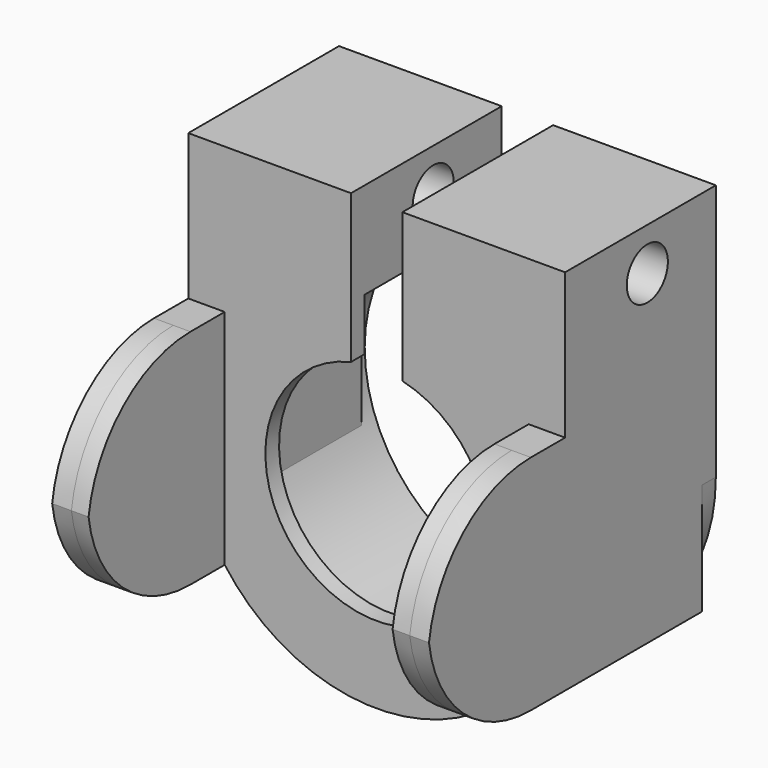
from build123d import *
from build123d import SkipClean  # not in build123d's __all__

# Parameters (mm, degrees)
F1_DEPTH    = 10
F3_D        = 3
F5_DEPTH    = 1
F6_W        = 2.1258803254
F6_H        = 13
F7_DEPTH    = 10
F8_T1_DEPTH = 39.6258803254
F8_T3_DEPTH = 39.6258803254


# Not quite as in the source:
# - a fillet or chamfer that OpenCascade refuses, or shapes differently, is made with other operations: its cross-section is extruded or revolved along the edge and cut away or added


with BuildPart() as f1:
    # F0 (on Front) → F1 (new body)
    with BuildSketch(Plane.XZ):
        with BuildLine():
            ThreePointArc((1.5, 9.3808315196), (0, -9.5), (-1.5, 9.3808315196))
            Line((-1.5, 9.3808315196), (-1.5, 15))
            Line((-1.5, 15), (-11, 15))
            Line((-11, 15), (-11, 0))
            ThreePointArc((-11, 0), (0, -11), (11, 0))
            Line((11, 0), (11, 15))
            Line((11, 15), (1.5, 15))
            Line((1.5, 15), (1.5, 9.3808315196))
        make_face()
    extrude(amount=F1_DEPTH)

    # F3 (through all)
    with Locations(Plane.YZ.offset(11)):
        with Locations((-5, 12.5)):
            Hole(F3_D / 2)

    # F4 (on face) → F5 (join)
    with BuildSketch(Plane.XZ.offset(10)):
        with BuildLine():
            Line((-1.5, 15), (-11, 15))
            Line((-11, 15), (-11, 0))
            ThreePointArc((-11, 0), (0, -11), (11, 0))
            Line((11, 0), (11, 15))
            Line((11, 15), (1.5, 15))
            Line((1.5, 15), (1.5, 6.3245553203))
            ThreePointArc((1.5, 6.3245553203), (0, -6.5), (-1.5, 6.3245553203))
            Line((-1.5, 6.3245553203), (-1.5, 15))
        make_face()
    extrude(amount=F5_DEPTH)

    # F6 (on face) → F7 (join, symmetric)
    with BuildSketch(Plane.XZ.offset(11)):
        with Locations((-9.9370598373, 0)):
            Rectangle(F6_W, F6_H)
        with Locations((9.9370598373, 0)):
            Rectangle(F6_W, F6_H)
    extrude(amount=F7_DEPTH, both=True)

    # F8: fillet of radius 7.5 on 4 edges, made by hand

    # F8_s2 → F8_t1 (cut)
    with BuildSketch(Plane.YZ.offset(-29.75)):
        with BuildLine():
            ThreePointArc((-13.5, -6.5), (-18.8033008589, -4.3033008589), (-21, 1))
            Line((-21, 1), (-21, -6.5))
            Line((-21, -6.5), (-13.5, -6.5))
        make_face()
        with BuildLine():
            ThreePointArc((-13.5, 6.5), (-18.8033008589, 4.3033008589), (-21, -1))
            Line((-21, -1), (-21, 6.5))
            Line((-21, 6.5), (-13.5, 6.5))
        make_face()
    extrude(amount=F8_T1_DEPTH, mode=Mode.SUBTRACT)

    # F8_s4 → F8_t3 (cut)
    with BuildSketch(Plane.YZ.offset(-9.8758803254)):
        with BuildLine():
            ThreePointArc((-21, -1), (-18.8033008589, 4.3033008589), (-13.5, 6.5))
            Line((-13.5, 6.5), (-21, 6.5))
            Line((-21, 6.5), (-21, -1))
        make_face()
        with BuildLine():
            ThreePointArc((-13.5, -6.5), (-18.8033008589, -4.3033008589), (-21, 1))
            Line((-21, 1), (-21, -6.5))
            Line((-21, -6.5), (-13.5, -6.5))
        make_face()
    with SkipClean():  # cleaning this boolean's faces spoils the solid; the shape is the same uncleaned
        extrude(amount=F8_T3_DEPTH, mode=Mode.SUBTRACT)


solid = f1.part
